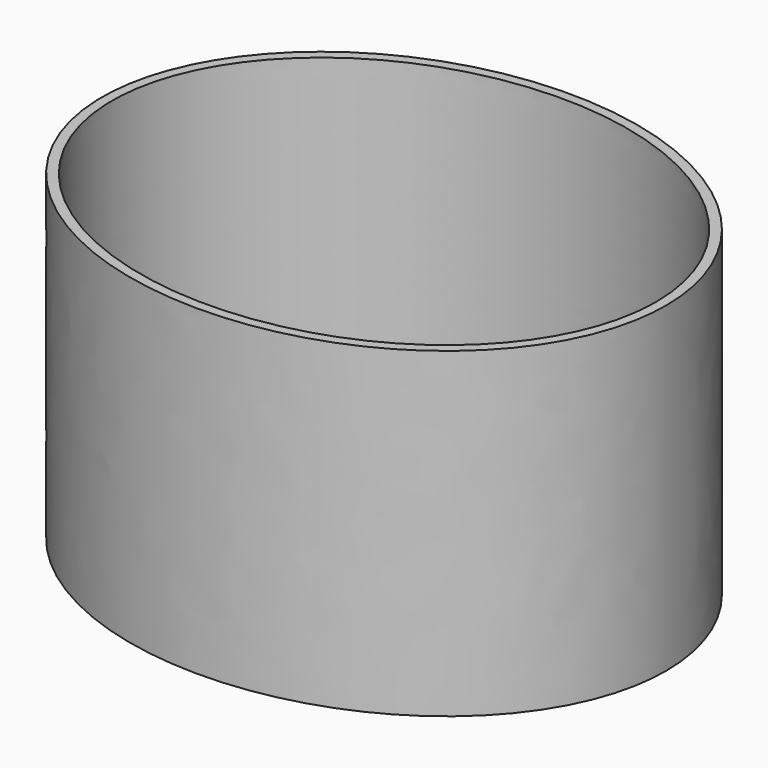
from build123d import *

# Parameters (mm, degrees)
F1_DEPTH = 65


# Not quite as in the source:
# - the dataset's text gives a spline's control points without its knots; the knots are read off the source's solid


with BuildPart() as f1:
    # F0 (on Top) → F1 (new body)
    with BuildSketch(Plane.XY):
        with BuildLine():
            add(Edge.make_bspline(
                [(57, 0), (57, 81.4063879557), (-28.5, 40.7031939779), (-114, 0), (-28.5, -40.7031939779), (57, -81.4063879557), (57, 0)],
                knots=[0, 0, 0, 2.0943951024, 2.0943951024, 4.1887902048, 4.1887902048, 6.2831853072, 6.2831853072, 6.2831853072], degree=2, weights=[1, 0.5, 1, 0.5, 1, 0.5, 1]))
        make_face()
        with BuildLine():
            add(Edge.make_bspline(
                [(55, 0), (55, 0.7377891856), (54.9555020967, 2.2133675567), (54.6909263921, 5.140941924), (54.0353522698, 8.7571398177), (52.7419533265, 12.9981758792), (50.9542178754, 17.1139839701), (48.6842415538, 21.0757211661), (45.9444133476, 24.8536730111), (43.279524691, 27.8239683429), (40.9262025744, 30.0769909931), (39.0490456845, 31.7038109634), (37.0739548603, 33.2534050521), (34.3325572315, 35.200369558), (30.7067612379, 37.4125685783), (26.0758083747, 39.6964826713), (21.2009303337, 41.5960045997), (16.1193711707, 43.097049238), (10.8687442099, 44.1860429537), (6.3828553591, 44.7391007643), (2.7484141768, 44.9624295594), (0, 45.0187852203), (-2.7484141768, 44.9624295594), (-6.3828553591, 44.7391007643), (-10.8687442099, 44.1860429537), (-16.1193711707, 43.097049238), (-21.2009303337, 41.5960045997), (-26.0758083747, 39.6964826713), (-30.7067612379, 37.4125685783), (-34.3325572315, 35.200369558), (-37.0739548603, 33.2534050521), (-39.0490456845, 31.7038109634), (-40.9262025744, 30.0769909931), (-43.279524691, 27.8239683429), (-45.9444133476, 24.8536730111), (-48.6842415538, 21.0757211661), (-50.9542178754, 17.1139839701), (-52.7419533265, 12.9981758792), (-54.0353522698, 8.7571398177), (-54.6909263921, 5.140941924), (-54.9555020967, 2.2133675567), (-55.0222489517, 0), (-54.9555020967, -2.2133675567), (-54.6909263921, -5.140941924), (-54.0353522698, -8.7571398177), (-52.7419533265, -12.9981758792), (-50.9542178754, -17.1139839701), (-48.6842415538, -21.0757211661), (-45.9444133476, -24.8536730111), (-43.279524691, -27.8239683429), (-40.9262025744, -30.0769909931), (-39.0490456845, -31.7038109634), (-37.0739548603, -33.2534050521), (-34.3325572315, -35.200369558), (-30.7067612379, -37.4125685783), (-26.0758083747, -39.6964826713), (-21.2009303337, -41.5960045997), (-16.1193711707, -43.097049238), (-10.8687442099, -44.1860429537), (-6.3828553591, -44.7391007643), (-2.7484141768, -44.9624295594), (0, -45.0187852203), (2.7484141768, -44.9624295594), (6.3828553591, -44.7391007643), (10.8687442099, -44.1860429537), (16.1193711707, -43.097049238), (21.2009303337, -41.5960045997), (26.0758083747, -39.6964826713), (30.7067612379, -37.4125685783), (34.3325572315, -35.200369558), (37.0739548603, -33.2534050521), (39.0490456845, -31.7038109634), (40.9262025744, -30.0769909931), (43.279524691, -27.8239683429), (45.9444133476, -24.8536730111), (48.6842415538, -21.0757211661), (50.9542178754, -17.1139839701), (52.7419533265, -12.9981758792), (54.0353522698, -8.7571398177), (54.6909263921, -5.140941924), (54.9555020967, -2.2133675567), (55, -0.7377891856), (55, 0)],
                knots=[0, 0, 0, 0, 0.0078125, 0.015625, 0.03125, 0.046875, 0.0625, 0.078125, 0.09375, 0.109375, 0.1171875, 0.125, 0.1328125, 0.140625, 0.15625, 0.171875, 0.1875, 0.203125, 0.21875, 0.234375, 0.2421875, 0.25, 0.2578125, 0.265625, 0.28125, 0.296875, 0.3125, 0.328125, 0.34375, 0.359375, 0.3671875, 0.375, 0.3828125, 0.390625, 0.40625, 0.421875, 0.4375, 0.453125, 0.46875, 0.484375, 0.4921875, 0.5, 0.5078125, 0.515625, 0.53125, 0.546875, 0.5625, 0.578125, 0.59375, 0.609375, 0.6171875, 0.625, 0.6328125, 0.640625, 0.65625, 0.671875, 0.6875, 0.703125, 0.71875, 0.734375, 0.7421875, 0.75, 0.7578125, 0.765625, 0.78125, 0.796875, 0.8125, 0.828125, 0.84375, 0.859375, 0.8671875, 0.875, 0.8828125, 0.890625, 0.90625, 0.921875, 0.9375, 0.953125, 0.96875, 0.984375, 0.9921875, 1, 1, 1, 1], degree=3))
        make_face(mode=Mode.SUBTRACT)
    extrude(amount=F1_DEPTH)


solid = f1.part
